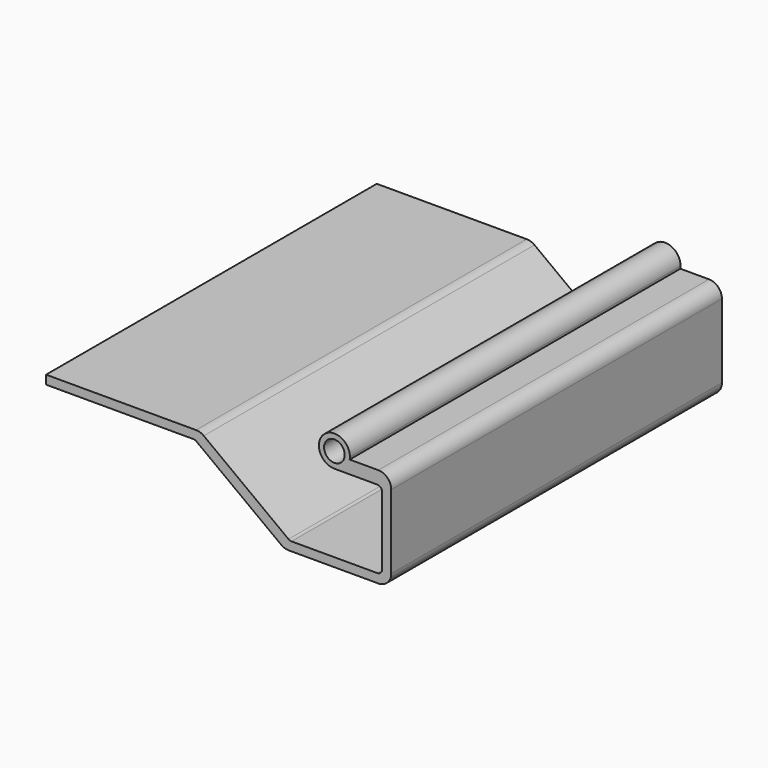
from build123d import *

# Parameters (mm, degrees)
F0_R     = 3.175
F1_DEPTH = 127
F2_R     = 3.9624
F3_R     = 1.524


# Not quite as in the source:
# - a feature names something its author has since deleted; it is built from what else it names


with BuildPart() as f1:
    # F0 (on Front) → F1 (new body)
    with BuildSketch(Plane.XZ):
        with BuildLine():
            ThreePointArc((4.7011447808, -0.762), (4.7471364141, -0.3822330647), (4.7625, 0))
            ThreePointArc((4.7625, 0), (-3.3675960454, 3.3675960454), (0, -4.7625))
            ThreePointArc((0, -4.7625), (3.0864527576, -3.6270119417), (4.7011447808, -0.762))
        make_face()
        Circle(F0_R, mode=Mode.SUBTRACT)
        with BuildLine():
            ThreePointArc((4.7011447808, -0.762), (3.0864527576, -3.6270119417), (0, -4.7625))
            Line((0, -4.7625), (14.6685, -4.7625))
            Line((14.6685, -4.7625), (14.6685, -28.702))
            Line((14.6685, -28.702), (-13.6858972215, -28.702))
            Line((-13.6858972215, -28.702), (-41.1854304771, -8.128))
            Line((-41.1854304771, -8.128), (-88.58598171, -8.128))
            Line((-88.58598171, -8.128), (-88.58598171, -10.83818))
            Line((-88.58598171, -10.83818), (-42.8310789114, -10.83818))
            Line((-42.8310789114, -10.83818), (-15.3315456557, -31.41218))
            Line((-15.3315456557, -31.41218), (17.4625, -31.41218))
            Line((17.4625, -31.41218), (17.4625, -0.762))
            Line((17.4625, -0.762), (4.7011447808, -0.762))
        make_face()
    extrude(amount=-F1_DEPTH)

    # F2
    f2_edges = [f1.edges().sort_by_distance(p)[0] for p in [
        (17.4625, 63.5, -0.762),
        (-15.331546, 63.5, -31.41218),
        (-41.18543, 63.5, -8.128),
        (17.4625, 63.5, -31.41218),
    ]]
    fillet(f2_edges, radius=F2_R)

    # F3
    f3_edges = [f1.edges().sort_by_distance(p)[0] for p in [
        (14.6685, 63.5, -4.7625),
        (-13.685897, 63.5, -28.702),
        (-42.831079, 63.5, -10.83818),
        (14.6685, 63.5, -28.702),
    ]]
    fillet(f3_edges, radius=F3_R)


solid = f1.part
